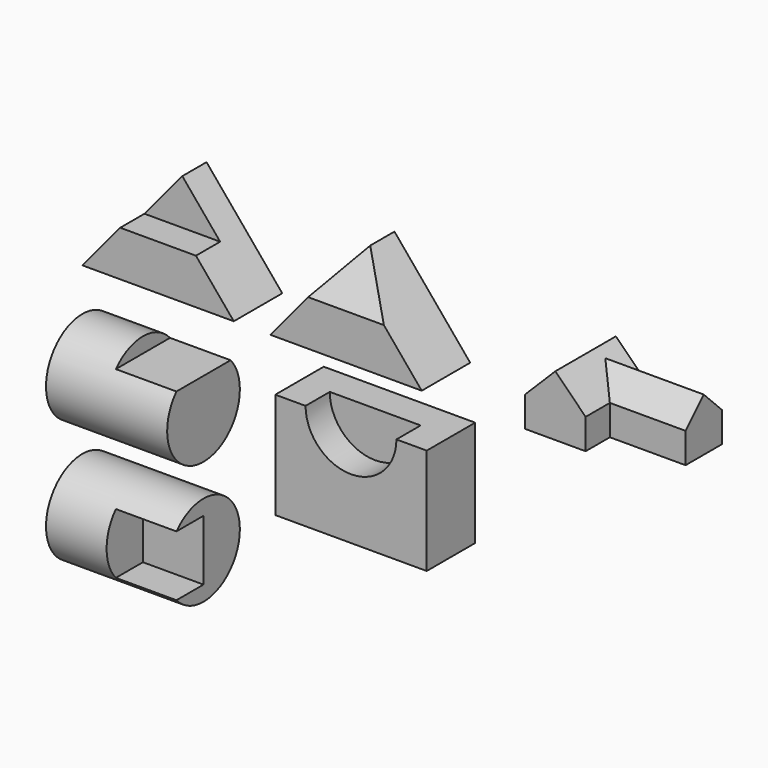
from build123d import *

# Parameters (mm, degrees)
F1_DEPTH  = 101.6
F3_DEPTH  = 50.8
F5_DEPTH  = 101.6
F9_DEPTH  = 70.612
F10_W     = 228.6
F10_H     = 101.6
F11_DEPTH = 127
F13_DEPTH = 139.7
F17_DEPTH = 50.8
F18_DEPTH = 127
F19_DEPTH = 177.8
F20_R     = 76.2
F21_DEPTH = 203.2
F23_DEPTH = 101.6
F24_R     = 76.2
F25_DEPTH = 203.2
F27_DEPTH = 101.6
F28_W     = 254
F28_H     = 177.8
F29_DEPTH = 101.6
F31_DEPTH = 50.8


with BuildPart() as f1:
    # F0 (on Front) → F1 (new body)
    with BuildSketch(Plane.XZ):
        Polygon((127, 152.4), (0, 0), (254, 0), align=None)
    extrude(amount=-F1_DEPTH)

    # F2 (on face) → F3 (cut)
    with BuildSketch(Plane.XZ):
        Polygon((63.5, 76.2), (127, 76.2), (190.5, 76.2), (127, 152.4), align=None)
    extrude(amount=-F3_DEPTH, mode=Mode.SUBTRACT)


with BuildPart() as f5:
    # F4 (on Front) → F5 (new body)
    with BuildSketch(Plane.XZ):
        Polygon((442.2074718067, 152.4), (315.2074718067, 0), (569.2074718067, 0), align=None)
    extrude(amount=-F5_DEPTH)

    # F8 (on face) → F9 (cut, symmetric)
    with BuildSketch(Plane.YZ.offset(442.2074718067)):
        Polygon((50.8, 152.4), (0, 152.4), (0, 76.2), align=None)
    extrude(amount=F9_DEPTH, both=True, mode=Mode.SUBTRACT)


with BuildPart() as f11:
    # F10 (on Front) → F11 (new body)
    with BuildSketch(Plane.XZ):
        with Locations((856.8012001758, 50.8)):
            Rectangle(F10_W, F10_H)
    extrude(amount=-F11_DEPTH)

    # F12 (on face) → F13 (cut)
    with BuildSketch(Plane.XZ):
        Polygon((844.1012001758, 101.6), (793.3012001758, 101.6), (844.1012001758, 50.8), align=None)
        Polygon((793.3012001758, 101.6), (742.5012001758, 101.6), (742.5012001758, 50.8), align=None)
    extrude(amount=-F13_DEPTH, mode=Mode.SUBTRACT)

    # F14 (on face) → F17 (cut)
    with BuildSketch(Plane.XZ):
        Polygon((844.1012001758, 101.6), (844.1012001758, 50.8), (844.1012001758, 0), (971.1012001758, 0), (971.1012001758, 50.8), (971.1012001758, 101.6), align=None)
    extrude(amount=-F17_DEPTH, mode=Mode.SUBTRACT)

    # F15 (on face) → F18 (cut)
    with BuildSketch(Plane.YZ.offset(971.1012001758)):
        Polygon((50.8, 0), (50.8, 50.8), (88.9, 88.9), (127, 50.8), (127, 101.6), (0, 101.6), (0, 0), align=None)
    extrude(amount=-F18_DEPTH, mode=Mode.SUBTRACT)

    # F16 (on face) → F19 (join)
    with BuildSketch(Plane.YZ.offset(971.1012001758)):
        Polygon((88.9, 88.9), (50.8, 50.8), (50.8, 0), (127, 0), (127, 50.8), align=None)
    extrude(amount=-F19_DEPTH)


with BuildPart() as f21:
    # F20 (on Right) → F21 (new body)
    with BuildSketch(Plane.YZ):
        with Locations((0, -147.8994190693)):
            Circle(F20_R)
    extrude(amount=F21_DEPTH)

    # F22 (on face) → F23 (cut)
    with BuildSketch(Plane.YZ.offset(203.2)):
        with BuildLine():
            Line((-56.7961266285, -97.0994190693), (0, -97.0994190693))
            Line((0, -97.0994190693), (56.7961266285, -97.0994190693))
            ThreePointArc((56.7961266285, -97.0994190693), (0, -71.6994190693), (-56.7961266285, -97.0994190693))
        make_face()
    extrude(amount=-F23_DEPTH, mode=Mode.SUBTRACT)


with BuildPart() as f25:
    # F24 (on Right) → F25 (new body)
    with BuildSketch(Plane.YZ):
        with Locations((0, -354.5046203547)):
            Circle(F24_R)
    extrude(amount=F25_DEPTH)

    # F26 (on face) → F27 (cut)
    with BuildSketch(Plane.YZ.offset(203.2)):
        with BuildLine():
            Line((0, -405.3046203547), (0, -354.5046203547))
            Line((0, -354.5046203547), (0, -303.7046203547))
            Line((0, -303.7046203547), (-56.7961266285, -303.7046203547))
            ThreePointArc((-56.7961266285, -303.7046203547), (-76.2, -354.5046203547), (-56.7961266285, -405.3046203547))
            Line((-56.7961266285, -405.3046203547), (0, -405.3046203547))
        make_face()
    extrude(amount=-F27_DEPTH, mode=Mode.SUBTRACT)


with BuildPart() as f29:
    # F28 (on Front) → F29 (new body)
    with BuildSketch(Plane.XZ):
        with Locations((450.5708919574, -174.6254190803)):
            Rectangle(F28_W, F28_H)
    extrude(amount=-F29_DEPTH)

    # F30 (on face) → F31 (cut)
    with BuildSketch(Plane.XZ):
        with BuildLine():
            ThreePointArc((374.3708919574, -85.7254190803), (450.5708919574, -161.9254190803), (526.7708919574, -85.7254190803))
            Line((526.7708919574, -85.7254190803), (374.3708919574, -85.7254190803))
        make_face()
    extrude(amount=-F31_DEPTH, mode=Mode.SUBTRACT)


solid = Compound([f1.part, f5.part, f11.part, f21.part, f25.part, f29.part])
